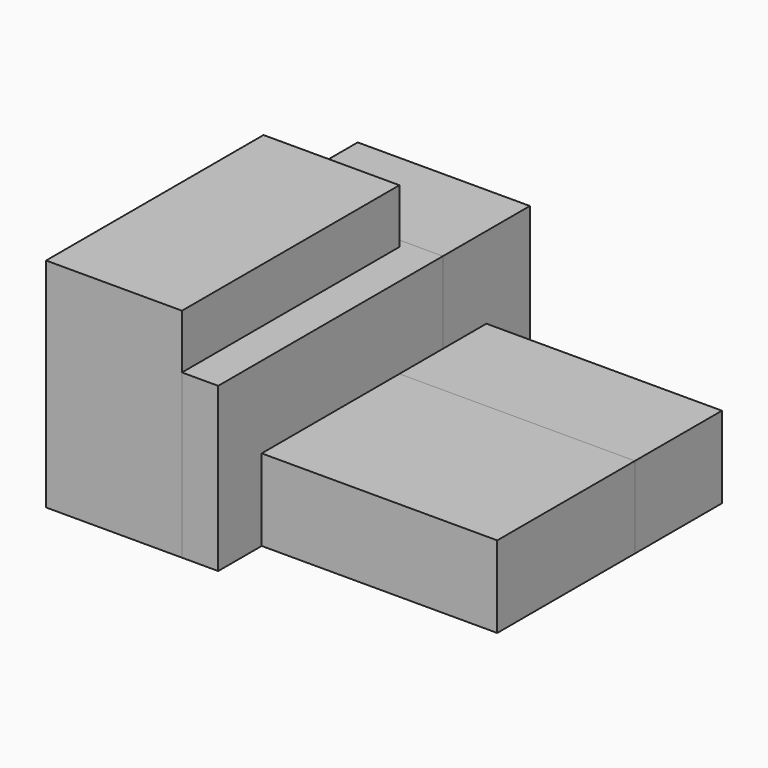
from build123d import *

# Parameters (mm, degrees)
F1_DEPTH = 914.4
F0_W     = 1320.8
F0_H     = 1574.8
F2_DEPTH = 457.2
F4_DEPTH = 914.4
F3_W     = 1320.8
F3_H     = 965.2
F5_DEPTH = 457.2
F6_W     = 762
F6_H     = 1524
F7_DEPTH = 1219.2


with BuildPart() as f1:
    # F0 (on Top) → F1 (new body)
    with BuildSketch(Plane.XY):
        Polygon((0, 2184.4), (0, 0), (965.2, 0), (965.2, 304.8), (965.2, 1879.6), (965.2, 2184.4), align=None)
    extrude(amount=F1_DEPTH)

    # F0 (on Top) → F2 (join)
    with BuildSketch(Plane.XY):
        with Locations((1625.6, 1092.2)):
            Rectangle(F0_W, F0_H)
    extrude(amount=F2_DEPTH)


with BuildPart() as f4:
    # F3 (on Top) → F4 (new body)
    with BuildSketch(Plane.XY):
        Polygon((0, 1574.8), (0, 0), (965.2, 0), (965.2, 304.8), (965.2, 1270), (965.2, 1574.8), align=None)
    extrude(amount=F4_DEPTH)

    # F3 (on Top) → F5 (join)
    with BuildSketch(Plane.XY):
        with Locations((1625.6, 787.4)):
            Rectangle(F3_W, F3_H)
    extrude(amount=F5_DEPTH)


with BuildPart() as f7:
    # F6 (on Top) → F7 (new body)
    with BuildSketch(Plane.XY):
        with Locations((381, 762)):
            Rectangle(F6_W, F6_H)
    extrude(amount=F7_DEPTH)


solid = Compound([f1.part, f4.part, f7.part])
